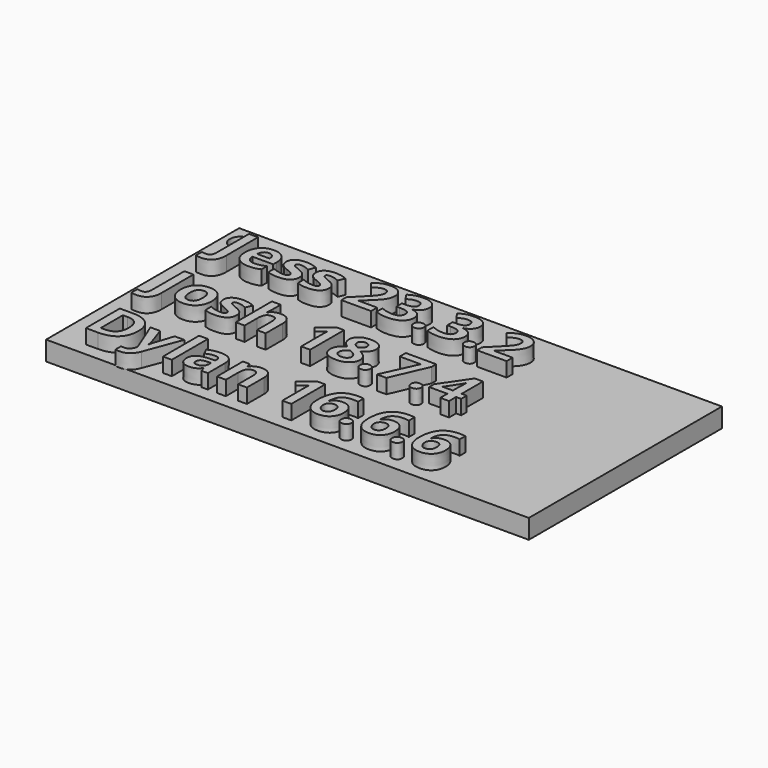
from build123d import *

# Parameters (mm, degrees)
F0_W         = 100
F0_H         = 50
F0_R         = 2.1724544303
F1_DEPTH     = 4
F2_TEXT_SIZE = 12.3026450687
F3_DEPTH     = 3


# Not quite as in the source:
# - Text() gives the source's letters only with a copy of the font that has no kerning and outlines rounded to 1/6400 em; it was checked with that copy


with BuildPart() as f1:
    # F0 (on Top) → F1 (new body)
    with BuildSketch(Plane.XY):
        Rectangle(F0_W, F0_H)
        with Locations((-46.6366000473, 21.1082473397)):
            Circle(F0_R, mode=Mode.SUBTRACT)
    extrude(amount=F1_DEPTH)

    # F2 (on face) → F3 (join)
    with BuildSketch(Plane.XY.offset(4)):
        with Locations((-45, 11.1420955505)):
            Text('Jess 23.3.2', F2_TEXT_SIZE, font='Open Sans', font_style=FontStyle.BOLD, text_align=(TextAlign.LEFT, TextAlign.BOTTOM))
        with Locations((-45, -5.5895017429)):
            Text('Josh 18.7.4', F2_TEXT_SIZE, font='Open Sans', font_style=FontStyle.BOLD, text_align=(TextAlign.LEFT, TextAlign.BOTTOM))
        with Locations((-45, -22.3210990363)):
            Text('Dylan 16.6.6', F2_TEXT_SIZE, font='Open Sans', font_style=FontStyle.BOLD, text_align=(TextAlign.LEFT, TextAlign.BOTTOM))
    extrude(amount=F3_DEPTH)


solid = f1.part
